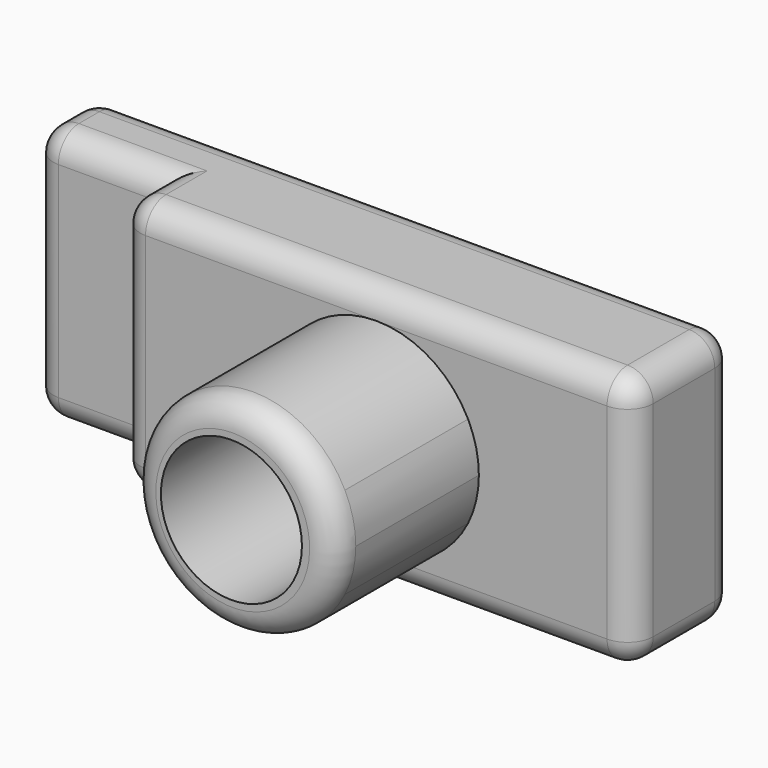
from build123d import *

# Parameters (mm, degrees)
F1_DEPTH     = 10
F3_DEPTH     = 7
F5_D         = 5.5
F6_T1_DEPTH  = 3
F6_T3_DEPTH  = 1
F6_T5_DEPTH  = 8
F6_T7_DEPTH  = 23
F6_T9_DEPTH  = 18
F6_T11_DEPTH = 4
F6_T13_DEPTH = 1
F6_S17_W     = 1
F6_S17_H     = 1
F6_T18_DEPTH = 1
F6_S23_W     = 1
F6_S23_H     = 1
F6_T24_DEPTH = 1
F6_S29_W     = 1
F6_S29_H     = 1
F6_T30_DEPTH = 1
F6_S35_W     = 1
F6_S35_H     = 1
F6_T36_DEPTH = 1
F6_S41_W     = 1
F6_S41_H     = 1
F6_T42_DEPTH = 1
F6_S47_W     = 1
F6_S47_H     = 1
F6_T48_DEPTH = 1
F6_S53_W     = 1
F6_S53_H     = 1
F6_T54_DEPTH = 1
F6_S59_W     = 1
F6_S59_H     = 1
F6_T60_DEPTH = 1
F6_S65_W     = 1
F6_S65_H     = 1
F6_T66_DEPTH = 1
F6_S71_W     = 1
F6_S71_H     = 1
F6_T72_DEPTH = 1
F6_T81_DEPTH = 6.5
F6_T85_DEPTH = 3.5
F6_T92_DEPTH = 6.5
F6_T96_DEPTH = 3.5


# Not quite as in the source:
# - a fillet or chamfer that OpenCascade refuses, or shapes differently, is made with other operations: its cross-section is extruded or revolved along the edge and cut away or added


with BuildPart() as f1:
    # F0 (on Top) → F1 (new body)
    with BuildSketch(Plane.XY):
        Polygon((-9.7338430583, 20.2614087611), (-34.7338430583, 20.2614087611), (-34.7338430583, 17.2614087611), (-29.7338430583, 17.2614087611), (-29.7338430583, 15.2614087611), (-9.7338430583, 15.2614087611), align=None)
    extrude(amount=F1_DEPTH)

    # F2 (on face) → F3 (join)
    with BuildSketch(Plane.XZ.offset(-15.2614087611)):
        with BuildLine():
            Line((-16.1561342943, 3.211145618), (-19.7338430583, 5))
            Line((-19.7338430583, 5), (-23.3115518223, 3.211145618))
            ThreePointArc((-23.3115518223, 3.211145618), (-19.7338430583, 1), (-16.1561342943, 3.211145618))
        make_face()
        with BuildLine():
            Line((-16.1561342943, 6.788854382), (-19.7338430583, 5))
            Line((-19.7338430583, 5), (-16.1561342943, 3.211145618))
            ThreePointArc((-16.1561342943, 3.211145618), (-15.8408471005, 4.0809883178), (-15.7338430583, 5))
            ThreePointArc((-15.7338430583, 5), (-15.8408471005, 5.9190116822), (-16.1561342943, 6.788854382))
        make_face()
        with BuildLine():
            ThreePointArc((-16.1561342943, 6.788854382), (-19.7338430583, 9), (-23.3115518223, 6.788854382))
            Line((-23.3115518223, 6.788854382), (-19.7338430583, 5))
            Line((-19.7338430583, 5), (-16.1561342943, 6.788854382))
        make_face()
        with BuildLine():
            Line((-19.7338430583, 5), (-23.3115518223, 6.788854382))
            ThreePointArc((-23.3115518223, 6.788854382), (-23.7338430583, 5), (-23.3115518223, 3.211145618))
            Line((-23.3115518223, 3.211145618), (-19.7338430583, 5))
        make_face()
    extrude(amount=F3_DEPTH)

    # F5 (through all)
    with Locations(Plane(origin=(0, 20.2614087611, 0), x_dir=(-1, 0, 0), z_dir=(0, 1, 0))):
        with Locations((19.7849275367, 4.9927774844)):
            Hole(F5_D / 2)

    # F6: fillet of radius 1 on 18 edges, made by hand

    # F6_s2 → F6_t1 (cut)
    with BuildSketch(Plane.XZ.offset(-19.2614087611)):
        with BuildLine():
            ThreePointArc((-9.7338430583, 9), (-10.0267362772, 9.7071067812), (-10.7338430583, 10))
            Line((-10.7338430583, 10), (-9.7338430583, 10))
            Line((-9.7338430583, 10), (-9.7338430583, 9))
        make_face()
        with BuildLine():
            ThreePointArc((-9.7338430583, 1), (-10.0267362772, 0.2928932188), (-10.7338430583, 0))
            Line((-10.7338430583, 0), (-9.7338430583, 0))
            Line((-9.7338430583, 0), (-9.7338430583, 1))
        make_face()
    extrude(amount=F6_T1_DEPTH, mode=Mode.SUBTRACT)

    # F6_s4 → F6_t3 (cut)
    with BuildSketch(Plane.XZ.offset(-19.2614087611)):
        with BuildLine():
            ThreePointArc((-33.7338430583, 10), (-34.4409498395, 9.7071067812), (-34.7338430583, 9))
            Line((-34.7338430583, 9), (-34.7338430583, 10))
            Line((-34.7338430583, 10), (-33.7338430583, 10))
        make_face()
        with BuildLine():
            ThreePointArc((-33.7338430583, 0), (-34.4409498395, 0.2928932188), (-34.7338430583, 1))
            Line((-34.7338430583, 1), (-34.7338430583, 0))
            Line((-34.7338430583, 0), (-33.7338430583, 0))
        make_face()
    extrude(amount=F6_T3_DEPTH, mode=Mode.SUBTRACT)

    # F6_s6 → F6_t5 (cut)
    with BuildSketch(Plane.XY.offset(1)):
        with BuildLine():
            ThreePointArc((-33.7338430583, 20.2614087611), (-34.4409498395, 19.9685155423), (-34.7338430583, 19.2614087611))
            Line((-34.7338430583, 19.2614087611), (-34.7338430583, 20.2614087611))
            Line((-34.7338430583, 20.2614087611), (-33.7338430583, 20.2614087611))
        make_face()
        with BuildLine():
            ThreePointArc((-34.7338430583, 18.2614087611), (-34.4409498395, 17.55430198), (-33.7338430583, 17.2614087611))
            Line((-33.7338430583, 17.2614087611), (-34.7338430583, 17.2614087611))
            Line((-34.7338430583, 17.2614087611), (-34.7338430583, 18.2614087611))
        make_face()
        with BuildLine():
            ThreePointArc((-10.7338430583, 20.2614087611), (-10.0267362772, 19.9685155423), (-9.7338430583, 19.2614087611))
            Line((-9.7338430583, 19.2614087611), (-9.7338430583, 20.2614087611))
            Line((-9.7338430583, 20.2614087611), (-10.7338430583, 20.2614087611))
        make_face()
        with BuildLine():
            ThreePointArc((-28.7338430583, 15.2614087611), (-29.4409498395, 15.55430198), (-29.7338430583, 16.2614087611))
            Line((-29.7338430583, 16.2614087611), (-29.7338430583, 15.2614087611))
            Line((-29.7338430583, 15.2614087611), (-28.7338430583, 15.2614087611))
        make_face()
        with BuildLine():
            ThreePointArc((-9.7338430583, 16.2614087611), (-10.0267362772, 15.55430198), (-10.7338430583, 15.2614087611))
            Line((-10.7338430583, 15.2614087611), (-9.7338430583, 15.2614087611))
            Line((-9.7338430583, 15.2614087611), (-9.7338430583, 16.2614087611))
        make_face()
    extrude(amount=F6_T5_DEPTH, mode=Mode.SUBTRACT)

    # F6_s8 → F6_t7 (cut)
    with BuildSketch(Plane.YZ.offset(-33.7338430583)):
        with BuildLine():
            ThreePointArc((20.2614087611, 1), (19.9685155423, 0.2928932188), (19.2614087611, 0))
            Line((19.2614087611, 0), (20.2614087611, 0))
            Line((20.2614087611, 0), (20.2614087611, 1))
        make_face()
        with BuildLine():
            ThreePointArc((20.2614087611, 9), (19.9685155423, 9.7071067812), (19.2614087611, 10))
            Line((19.2614087611, 10), (20.2614087611, 10))
            Line((20.2614087611, 10), (20.2614087611, 9))
        make_face()
    extrude(amount=F6_T7_DEPTH, mode=Mode.SUBTRACT)

    # F6_s10 → F6_t9 (cut)
    with BuildSketch(Plane.YZ.offset(-28.7338430583)):
        with BuildLine():
            ThreePointArc((16.2614087611, 0), (15.55430198, 0.2928932188), (15.2614087611, 1))
            Line((15.2614087611, 1), (15.2614087611, 0))
            Line((15.2614087611, 0), (16.2614087611, 0))
        make_face()
        with BuildLine():
            ThreePointArc((16.2614087611, 10), (15.55430198, 9.7071067812), (15.2614087611, 9))
            Line((15.2614087611, 9), (15.2614087611, 10))
            Line((15.2614087611, 10), (16.2614087611, 10))
        make_face()
    extrude(amount=F6_T9_DEPTH, mode=Mode.SUBTRACT)

    # F6_s12 → F6_t11 (cut)
    with BuildSketch(Plane.YZ.offset(-33.7338430583)):
        with BuildLine():
            ThreePointArc((18.2614087611, 0), (17.55430198, 0.2928932188), (17.2614087611, 1))
            Line((17.2614087611, 1), (17.2614087611, 0))
            Line((17.2614087611, 0), (18.2614087611, 0))
        make_face()
        with BuildLine():
            ThreePointArc((18.2614087611, 10), (17.55430198, 9.7071067812), (17.2614087611, 9))
            Line((17.2614087611, 9), (17.2614087611, 10))
            Line((17.2614087611, 10), (18.2614087611, 10))
        make_face()
    extrude(amount=F6_T11_DEPTH, mode=Mode.SUBTRACT)

    # F6_s14 → F6_t13 (cut)
    with BuildSketch(Plane.XZ.offset(-17.2614087611)):
        with BuildLine():
            ThreePointArc((-28.7338430583, 0), (-29.4409498395, 0.2928932188), (-29.7338430583, 1))
            Line((-29.7338430583, 1), (-29.7338430583, 0))
            Line((-29.7338430583, 0), (-28.7338430583, 0))
        make_face()
        with BuildLine():
            ThreePointArc((-28.7338430583, 10), (-29.4409498395, 9.7071067812), (-29.7338430583, 9))
            Line((-29.7338430583, 9), (-29.7338430583, 10))
            Line((-29.7338430583, 10), (-28.7338430583, 10))
        make_face()
    extrude(amount=F6_T13_DEPTH, mode=Mode.SUBTRACT)


with BuildPart() as f6_tool16:
    # F6_s17 → F6_t18 (new body)
    with BuildSketch(Plane.YZ.offset(-10.7338430583)):
        with Locations((15.7614087611, 9.5)):
            Rectangle(F6_S17_W, F6_S17_H)
    extrude(amount=F6_T18_DEPTH)

    # F6_s19 → F6_t20 (revolve, cut)
    with BuildSketch(Plane(origin=(-10.7338430583, 16.2614087611, 9), x_dir=(0, 0.7071067812, -0.7071067812), z_dir=(0, -0.7071067812, -0.7071067812))):
        with BuildLine():
            ThreePointArc((0, -1), (1, 0), (0, 1))
            Line((0, 1), (0, -1))
        make_face()
    revolve(axis=Axis((-10.7338430583, 16.2614087611, 9), (1, 0, 0)), mode=Mode.SUBTRACT)


with BuildPart() as f1_1:
    add(f1.part)

    # F6_t15: cut F6_tool16
    add(f6_tool16.part, mode=Mode.SUBTRACT)


with BuildPart() as f6_tool22:
    # F6_s23 → F6_t24 (new body)
    with BuildSketch(Plane.XZ.offset(-19.2614087611)):
        with Locations((-10.2338430583, 9.5)):
            Rectangle(F6_S23_W, F6_S23_H)
    extrude(amount=-F6_T24_DEPTH)

    # F6_s25 → F6_t26 (revolve, cut)
    with BuildSketch(Plane(origin=(-10.7338430583, 19.2614087611, 9), x_dir=(-0.7071067812, 0, -0.7071067812), z_dir=(0.7071067812, 0, -0.7071067812))):
        with BuildLine():
            ThreePointArc((0, -1), (1, 0), (0, 1))
            Line((0, 1), (0, -1))
        make_face()
    revolve(axis=Axis((-10.7338430583, 19.2614087611, 9), (0, 1, 0)), mode=Mode.SUBTRACT)


with BuildPart() as f1_2:
    add(f1_1.part)

    # F6_t21: cut F6_tool22
    add(f6_tool22.part, mode=Mode.SUBTRACT)


with BuildPart() as f6_tool28:
    # F6_s29 → F6_t30 (new body)
    with BuildSketch(Plane.YZ.offset(-10.7338430583)):
        with Locations((15.7614087611, 0.5)):
            Rectangle(F6_S29_W, F6_S29_H)
    extrude(amount=F6_T30_DEPTH)

    # F6_s31 → F6_t32 (revolve, cut)
    with BuildSketch(Plane(origin=(-10.7338430583, 16.2614087611, 1), x_dir=(0, 0.7071067812, 0.7071067812), z_dir=(0, 0.7071067812, -0.7071067812))):
        with BuildLine():
            ThreePointArc((0, -1), (1, 0), (0, 1))
            Line((0, 1), (0, -1))
        make_face()
    revolve(axis=Axis((-10.7338430583, 16.2614087611, 1), (1, 0, 0)), mode=Mode.SUBTRACT)


with BuildPart() as f1_3:
    add(f1_2.part)

    # F6_t27: cut F6_tool28
    add(f6_tool28.part, mode=Mode.SUBTRACT)


with BuildPart() as f6_tool34:
    # F6_s35 → F6_t36 (new body)
    with BuildSketch(Plane.XZ.offset(-19.2614087611)):
        with Locations((-10.2338430583, 0.5)):
            Rectangle(F6_S35_W, F6_S35_H)
    extrude(amount=-F6_T36_DEPTH)

    # F6_s37 → F6_t38 (revolve, cut)
    with BuildSketch(Plane(origin=(-10.7338430583, 19.2614087611, 1), x_dir=(-0.7071067812, 0, 0.7071067812), z_dir=(-0.7071067812, 0, -0.7071067812))):
        with BuildLine():
            ThreePointArc((0, -1), (1, 0), (0, 1))
            Line((0, 1), (0, -1))
        make_face()
    revolve(axis=Axis((-10.7338430583, 19.2614087611, 1), (0, 1, 0)), mode=Mode.SUBTRACT)


with BuildPart() as f1_4:
    add(f1_3.part)

    # F6_t33: cut F6_tool34
    add(f6_tool34.part, mode=Mode.SUBTRACT)


with BuildPart() as f6_tool40:
    # F6_s41 → F6_t42 (new body)
    with BuildSketch(Plane.XZ.offset(-19.2614087611)):
        with Locations((-34.2338430583, 9.5)):
            Rectangle(F6_S41_W, F6_S41_H)
    extrude(amount=-F6_T42_DEPTH)

    # F6_s43 → F6_t44 (revolve, cut)
    with BuildSketch(Plane(origin=(-33.7338430583, 19.2614087611, 9), x_dir=(0.7071067812, 0, -0.7071067812), z_dir=(0.7071067812, 0, 0.7071067812))):
        with BuildLine():
            ThreePointArc((0, -1), (1, 0), (0, 1))
            Line((0, 1), (0, -1))
        make_face()
    revolve(axis=Axis((-33.7338430583, 19.2614087611, 9), (0, 1, 0)), mode=Mode.SUBTRACT)


with BuildPart() as f1_5:
    add(f1_4.part)

    # F6_t39: cut F6_tool40
    add(f6_tool40.part, mode=Mode.SUBTRACT)


with BuildPart() as f6_tool46:
    # F6_s47 → F6_t48 (new body)
    with BuildSketch(Plane.XY.offset(9)):
        with Locations((-34.2338430583, 17.7614087611)):
            Rectangle(F6_S47_W, F6_S47_H)
    extrude(amount=F6_T48_DEPTH)

    # F6_s49 → F6_t50 (revolve, cut)
    with BuildSketch(Plane(origin=(-33.7338430583, 18.2614087611, 9), x_dir=(0.7071067812, 0.7071067812, 0), z_dir=(0.7071067812, -0.7071067812, 0))):
        with BuildLine():
            ThreePointArc((0, -1), (1, 0), (0, 1))
            Line((0, 1), (0, -1))
        make_face()
    revolve(axis=Axis((-33.7338430583, 18.2614087611, 9), (0, 0, 1)), mode=Mode.SUBTRACT)


with BuildPart() as f1_6:
    add(f1_5.part)

    # F6_t45: cut F6_tool46
    add(f6_tool46.part, mode=Mode.SUBTRACT)


with BuildPart() as f6_tool52:
    # F6_s53 → F6_t54 (new body)
    with BuildSketch(Plane.XZ.offset(-19.2614087611)):
        with Locations((-34.2338430583, 0.5)):
            Rectangle(F6_S53_W, F6_S53_H)
    extrude(amount=-F6_T54_DEPTH)

    # F6_s55 → F6_t56 (revolve, cut)
    with BuildSketch(Plane(origin=(-33.7338430583, 19.2614087611, 1), x_dir=(0.7071067812, 0, 0.7071067812), z_dir=(-0.7071067812, 0, 0.7071067812))):
        with BuildLine():
            ThreePointArc((0, -1), (1, 0), (0, 1))
            Line((0, 1), (0, -1))
        make_face()
    revolve(axis=Axis((-33.7338430583, 19.2614087611, 1), (0, 1, 0)), mode=Mode.SUBTRACT)


with BuildPart() as f1_7:
    add(f1_6.part)

    # F6_t51: cut F6_tool52
    add(f6_tool52.part, mode=Mode.SUBTRACT)


with BuildPart() as f6_tool58:
    # F6_s59 → F6_t60 (new body)
    with BuildSketch(Plane.XY.offset(1)):
        with Locations((-34.2338430583, 17.7614087611)):
            Rectangle(F6_S59_W, F6_S59_H)
    extrude(amount=-F6_T60_DEPTH)

    # F6_s61 → F6_t62 (revolve, cut)
    with BuildSketch(Plane(origin=(-33.7338430583, 18.2614087611, 1), x_dir=(0.7071067812, 0.7071067812, 0), z_dir=(-0.7071067812, 0.7071067812, 0))):
        with BuildLine():
            ThreePointArc((0, -1), (1, 0), (0, 1))
            Line((0, 1), (0, -1))
        make_face()
    revolve(axis=Axis((-33.7338430583, 18.2614087611, 1), (0, 0, -1)), mode=Mode.SUBTRACT)


with BuildPart() as f1_8:
    add(f1_7.part)

    # F6_t57: cut F6_tool58
    add(f6_tool58.part, mode=Mode.SUBTRACT)


with BuildPart() as f6_tool64:
    # F6_s65 → F6_t66 (new body)
    with BuildSketch(Plane.YZ.offset(-28.7338430583)):
        with Locations((15.7614087611, 0.5)):
            Rectangle(F6_S65_W, F6_S65_H)
    extrude(amount=-F6_T66_DEPTH)

    # F6_s67 → F6_t68 (revolve, cut)
    with BuildSketch(Plane(origin=(-28.7338430583, 16.2614087611, 1), x_dir=(0, 0.7071067812, 0.7071067812), z_dir=(0, -0.7071067812, 0.7071067812))):
        with BuildLine():
            ThreePointArc((0, -1), (1, 0), (0, 1))
            Line((0, 1), (0, -1))
        make_face()
    revolve(axis=Axis((-28.7338430583, 16.2614087611, 1), (-1, 0, 0)), mode=Mode.SUBTRACT)


with BuildPart() as f1_9:
    add(f1_8.part)

    # F6_t63: cut F6_tool64
    add(f6_tool64.part, mode=Mode.SUBTRACT)


with BuildPart() as f6_tool70:
    # F6_s71 → F6_t72 (new body)
    with BuildSketch(Plane.YZ.offset(-28.7338430583)):
        with Locations((15.7614087611, 9.5)):
            Rectangle(F6_S71_W, F6_S71_H)
    extrude(amount=-F6_T72_DEPTH)

    # F6_s73 → F6_t74 (revolve, cut)
    with BuildSketch(Plane(origin=(-28.7338430583, 16.2614087611, 9), x_dir=(0, 0.7071067812, -0.7071067812), z_dir=(0, 0.7071067812, 0.7071067812))):
        with BuildLine():
            ThreePointArc((0, -1), (1, 0), (0, 1))
            Line((0, 1), (0, -1))
        make_face()
    revolve(axis=Axis((-28.7338430583, 16.2614087611, 9), (-1, 0, 0)), mode=Mode.SUBTRACT)


with BuildPart() as f1_10:
    add(f1_9.part)

    # F6_t69: cut F6_tool70
    add(f6_tool70.part, mode=Mode.SUBTRACT)

    # F6_s75 → F6_t76 (revolve, cut)
    with BuildSketch(Plane(origin=(-1.9467686117, 0, -3.8935372233), x_dir=(0, 1, 0), z_dir=(0.4472135955, 0, 0.894427191))):
        with BuildLine():
            ThreePointArc((8.2614087611, 22.8865537918), (8.55430198, 23.593660573), (9.2614087611, 23.8865537918))
            Line((9.2614087611, 23.8865537918), (8.2614087611, 23.8865537918))
            Line((8.2614087611, 23.8865537918), (8.2614087611, 22.8865537918))
        make_face()
    revolve(axis=Axis((-19.7338430583, 8.2614087611, 5), (0, -1, 0)), mode=Mode.SUBTRACT)


with BuildPart() as f6_tool79:
    # F6_s80 → F6_t81 (new body)
    with BuildSketch(Plane.YZ.offset(-33.7338430583)):
        with BuildLine():
            ThreePointArc((18.2614087611, 0), (17.55430198, 0.2928932188), (17.2614087611, 1))
            Line((17.2614087611, 1), (17.2614087611, 0))
            Line((17.2614087611, 0), (18.2614087611, 0))
        make_face()
    extrude(amount=F6_T81_DEPTH)

    split(bisect_by=Plane.YZ.offset(-29.7338430583), keep=Keep.TOP)


with BuildPart() as f6_tool83:
    # F6_s84 → F6_t85 (new body)
    with BuildSketch(Plane.XZ.offset(-19.7614087611)):
        with BuildLine():
            ThreePointArc((-28.7338430583, 0), (-29.4409498395, 0.2928932188), (-29.7338430583, 1))
            Line((-29.7338430583, 1), (-29.7338430583, 0))
            Line((-29.7338430583, 0), (-28.7338430583, 0))
        make_face()
    extrude(amount=F6_T85_DEPTH)

    split(bisect_by=Plane.XZ.offset(-17.2614087611), keep=Keep.BOTTOM)


with BuildPart() as f6_tool79_1:
    add(f6_tool79.part)

    # F6_t87: intersect F6_tool83
    add(f6_tool83.part, mode=Mode.INTERSECT)


with BuildPart() as f1_11:
    add(f1_10.part)

    # F6_t77: cut F6_tool79
    add(f6_tool79_1.part, mode=Mode.SUBTRACT)


with BuildPart() as f6_tool90:
    # F6_s91 → F6_t92 (new body)
    with BuildSketch(Plane.YZ.offset(-33.7338430583)):
        with BuildLine():
            ThreePointArc((18.2614087611, 10), (17.55430198, 9.7071067812), (17.2614087611, 9))
            Line((17.2614087611, 9), (17.2614087611, 10))
            Line((17.2614087611, 10), (18.2614087611, 10))
        make_face()
    extrude(amount=F6_T92_DEPTH)

    split(bisect_by=Plane.YZ.offset(-29.7338430583), keep=Keep.TOP)


with BuildPart() as f6_tool94:
    # F6_s95 → F6_t96 (new body)
    with BuildSketch(Plane.XZ.offset(-19.7614087611)):
        with BuildLine():
            ThreePointArc((-28.7338430583, 10), (-29.4409498395, 9.7071067812), (-29.7338430583, 9))
            Line((-29.7338430583, 9), (-29.7338430583, 10))
            Line((-29.7338430583, 10), (-28.7338430583, 10))
        make_face()
    extrude(amount=F6_T96_DEPTH)

    split(bisect_by=Plane.XZ.offset(-17.2614087611), keep=Keep.BOTTOM)


with BuildPart() as f6_tool90_1:
    add(f6_tool90.part)

    # F6_t98: intersect F6_tool94
    add(f6_tool94.part, mode=Mode.INTERSECT)


with BuildPart() as f1_12:
    add(f1_11.part)

    # F6_t88: cut F6_tool90
    add(f6_tool90_1.part, mode=Mode.SUBTRACT)


solid = f1_12.part
